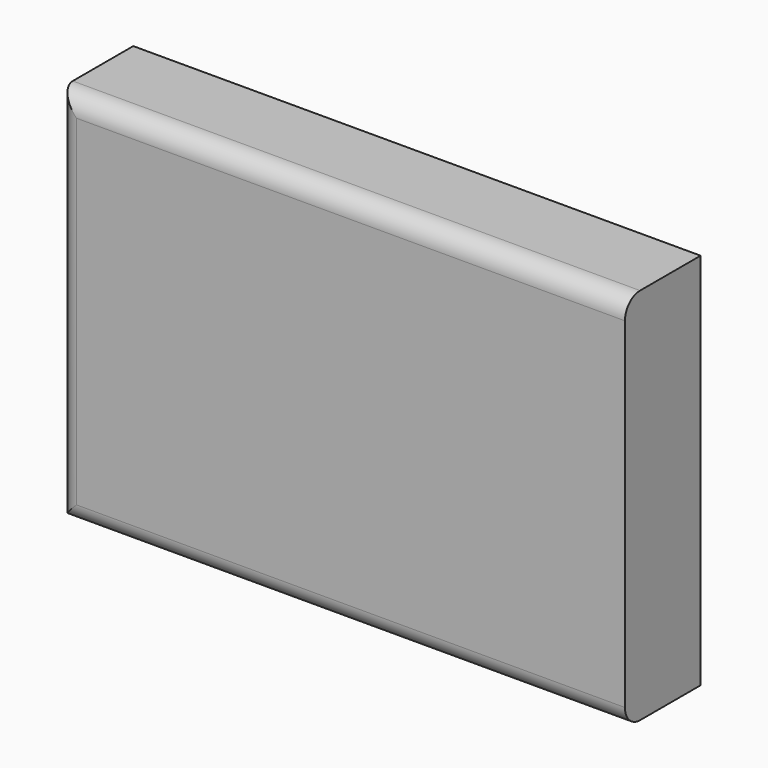
from build123d import *

# Parameters (mm, degrees)
F0_W     = 150
F0_H     = 100
F1_DEPTH = 25
F2_R     = 5


# Not quite as in the source:
# - a feature names something its author has since deleted; it is built from what else it names


with BuildPart() as f1:
    # F0 (on Front) → F1 (new body)
    with BuildSketch(Plane.XZ):
        with Locations((8.1972908229, 0)):
            Rectangle(F0_W, F0_H)
    extrude(amount=F1_DEPTH)

    # F2
    f2_edges = [f1.edges().sort_by_distance(p)[0] for p in [
        (8.197291, -25, 50),
        (-66.802709, -25, 0),
        (8.197291, -25, -50),
    ]]
    fillet(f2_edges, radius=F2_R)


solid = f1.part
